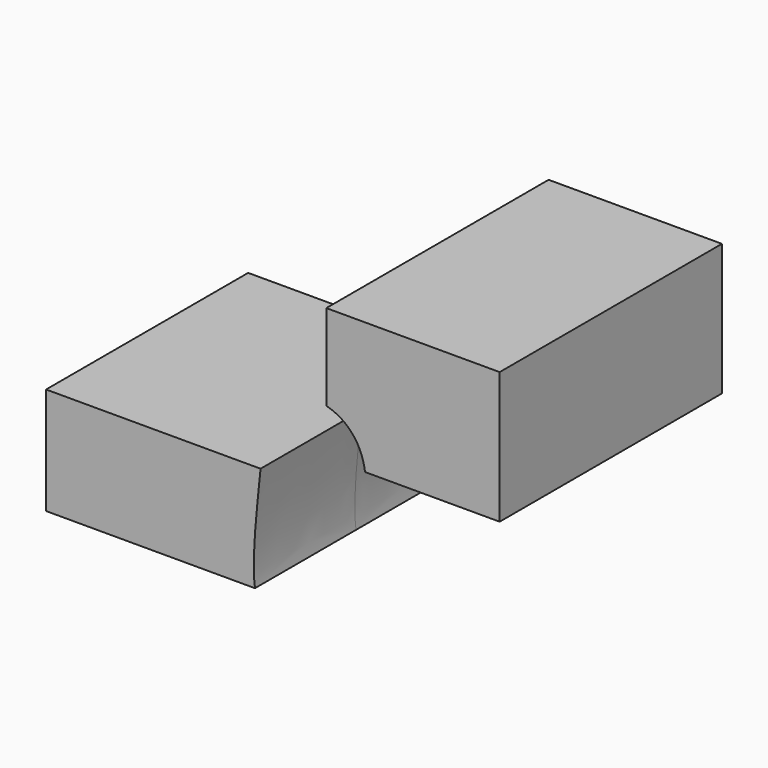
from build123d import *

# Parameters (mm, degrees)
F1_DEPTH = 63.5
F2_DEPTH = 12.7


# Not quite as in the source:
# - the dataset's text gives a spline's control points without its knots; the knots are read off the source's solid


with BuildPart() as f1:
    # F0 (on Front) → F1 (new body, symmetric)
    with BuildSketch(Plane.XZ):
        with BuildLine():
            Line((44.3445303026, 26.9082457591), (-63.5, 26.9082457591))
            Line((-63.5, 26.9082457591), (-63.5, -26.9082457591))
            Line((-63.5, -26.9082457591), (41.5330206736, -26.9082457591))
            add(Edge.make_bspline(
                [(41.5330206736, -26.9082457591), (41.5206891704, -26.8319854492), (41.3448448448, -25.7230965065), (41.1156345492, -23.6997117475), (40.9438322264, -20.8519320576), (40.881307, -17.9705748006), (40.9019094918, -14.997119488), (40.9913966742, -11.9042433146), (41.1401351146, -8.6814153594), (41.3407956994, -5.32812682), (41.6692584128, -0.6908531378), (42.1797414921, 5.3943561937), (42.9095362254, 13.0529659742), (43.6478674391, 20.2794962315), (44.1353924709, 24.9222708035), (44.3445303026, 26.9082457591)],
                knots=[0.7488512035, 0.7488512035, 0.7488512035, 0.7488512035, 0.75, 0.765625, 0.78125, 0.796875, 0.8125, 0.828125, 0.84375, 0.859375, 0.875, 0.90625, 0.9375, 0.96875, 0.9921519733, 0.9921519733, 0.9921519733, 0.9921519733], degree=3))
        make_face()
    extrude(amount=F1_DEPTH, both=True)


with BuildPart() as f1b:
    # F0 (on Front) → F1, piece 2 (new body, symmetric)
    with BuildSketch(Plane.XZ):
        with BuildLine():
            add(Edge.make_bspline(
                [(87.5728937206, 73.9479044282), (88.1080690446, 73.8133450078), (89.4580280251, 73.430626286), (91.6770203646, 72.6026408552), (94.1885548405, 71.3450272992), (96.6360890257, 69.7449658053), (98.9231882342, 67.8241603771), (100.9632190462, 65.6409923948), (102.6986997876, 63.2785305227), (104.109828379, 60.8228273116), (105.2096171996, 58.3492731764), (106.0320355859, 55.8959300691), (106.5976249855, 53.5973499201), (106.8784564156, 51.9945597192), (106.99856399, 51.1413742955), (107.0180190242, 50.9972441844)],
                knots=[0.158799995, 0.158799995, 0.158799995, 0.158799995, 0.1640625, 0.171875, 0.1796875, 0.1875, 0.1953125, 0.203125, 0.2109375, 0.21875, 0.2265625, 0.234375, 0.2421875, 0.25, 0.2515962027, 0.2515962027, 0.2515962027, 0.2515962027], degree=3))
            Line((107.0180190242, 50.9972441844), (174.7305428356, 50.9972441844))
            Line((174.7305428356, 50.9972441844), (174.7305428356, 117.2363148355))
            Line((174.7305428356, 117.2363148355), (87.5728937206, 117.2363148355))
            Line((87.5728937206, 117.2363148355), (87.5728937206, 73.9479044282))
        make_face()
    extrude(amount=F1_DEPTH, both=True)

    # F2 (add, symmetric): a face of the model
    f2_faces = [f1b.faces().sort_by_distance(p)[0] for p in [
        (133.2489364203, -63.5, 85.5209468782),
    ]]
    extrude(f2_faces, amount=F2_DEPTH, both=True)


solid = Compound([f1.part, f1b.part])
